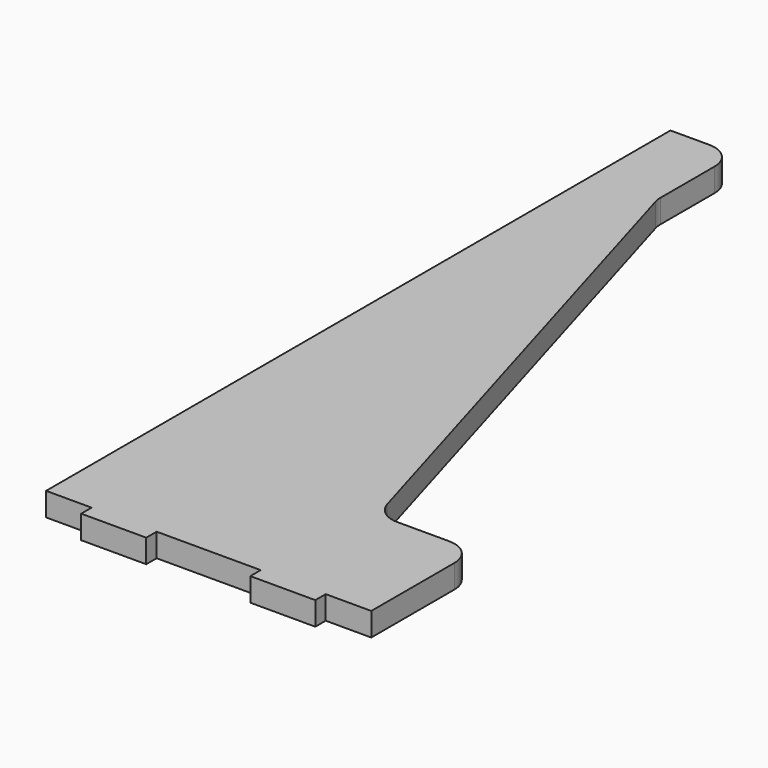
from build123d import *

# Parameters (mm, degrees)
F1_DEPTH = 18
F3_DEPTH = 25
F4_R     = 20


with BuildPart() as f1:
    # F0 (on Top) → F1 (new body)
    with BuildSketch(Plane.XY):
        Polygon((158.1674836576, 528.3263906837), (-91.8325163424, 528.3263906837), (-91.8325163424, -71.6736093163), (-56.8325163424, -71.6736093163), (-56.8325163424, -81.6736093163), (-6.8325163424, -81.6736093163), (-6.8325163424, -71.6736093163), (73.1674836576, -71.6736093163), (73.1674836576, -81.6736093163), (123.1674836576, -81.6736093163), (123.1674836576, -71.6736093163), (158.1674836576, -71.6736093163), align=None)
    extrude(amount=F1_DEPTH)

    # F2 (on face) → F3 (cut)
    with BuildSketch(Plane.XY.offset(18)):
        Polygon((158.1674836576, 528.3263906837), (-41.8325163424, 528.3263906837), (-41.8325163424, 453.3263906837), (83.1674836576, 28.3263906837), (158.1674836576, 28.3263906837), align=None)
    extrude(amount=-F3_DEPTH, mode=Mode.SUBTRACT)

    # F4
    f4_edges = [f1.edges().sort_by_distance(p)[0] for p in [
        (-41.832516, 528.326391, 9),
        (158.167484, 28.326391, 9),
        (-41.832516, 453.326391, 9),
        (83.167484, 28.326391, 9),
    ]]
    fillet(f4_edges, radius=F4_R)


solid = f1.part
